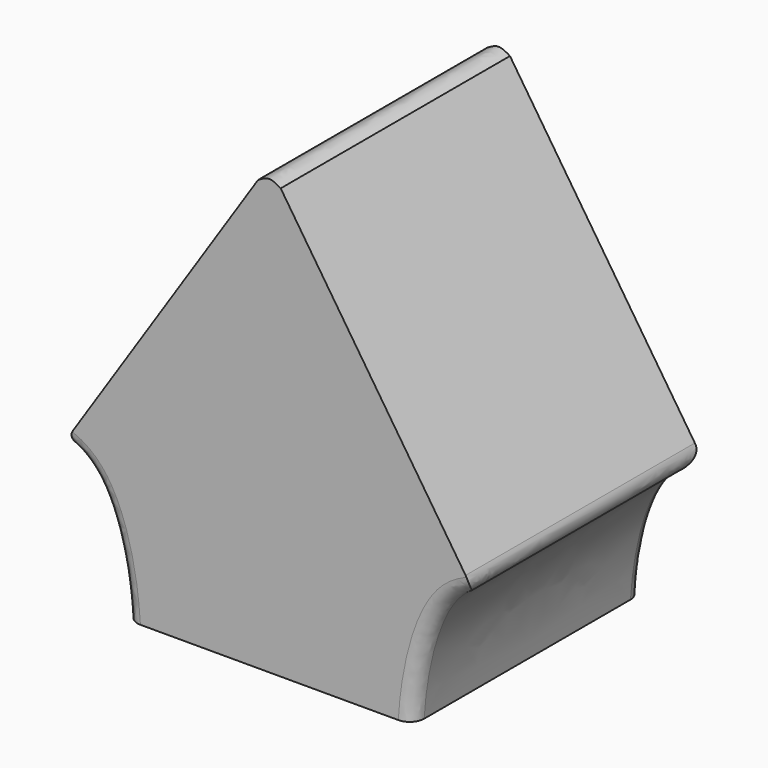
from build123d import *

# Parameters (mm, degrees)
F1_DEPTH = 20
F2_R     = 1


# Not quite as in the source:
# - a feature names something its author has since deleted; it is built from what else it names


with BuildPart() as f1:
    # F0 (on Front) → F1 (new body)
    with BuildSketch(Plane.XZ):
        with BuildLine():
            add(Edge.make_bspline(
                [(-14.320673421, 9.4697382301), (-13.2394510975, 9.0805694331), (-11.3333298848, 7.4710466695), (-10.1861008598, 3.0568630532), (-10, 0)],
                knots=[0, 0, 0, 0, 0.3950023229, 1, 1, 1, 1], degree=3))
            Line((-10, 0), (0, 0))
            Line((0, 0), (10, 0))
            add(Edge.make_bspline(
                [(14.320673421, 9.4697382301), (13.2394510975, 9.0805694331), (11.3333298848, 7.4710466695), (10.1861008598, 3.0568630532), (10, 0)],
                knots=[0, 0, 0, 0, 0.3950023229, 1, 1, 1, 1], degree=3))
            Line((14.320673421, 9.4697382301), (0.7904520571, 30))
            add(Edge.make_bspline(
                [(-0.7904520571, 30), (-0.5269680381, 30.1565037668), (0, 30.4695113003), (0.5269680381, 30.1565037668), (0.7904520571, 30)],
                knots=[0, 0, 0, 0, 0.5, 1, 1, 1, 1], degree=3))
            Line((-0.7904520571, 30), (-14.320673421, 9.4697382301))
        make_face()
    extrude(amount=F1_DEPTH)

    # F2
    f2_edges = [f1.edges().sort_by_distance(p)[0] for p in [
        (-14.320673, -10, 9.469738),
        (14.320673, -10, 9.469738),
        (-10.973556, 0, 5.385962),
        (-10.973556, -20, 5.385962),
        (10.973556, 0, 5.385962),
        (10.973556, -20, 5.385962),
    ]]
    fillet(f2_edges, radius=F2_R)


solid = f1.part
